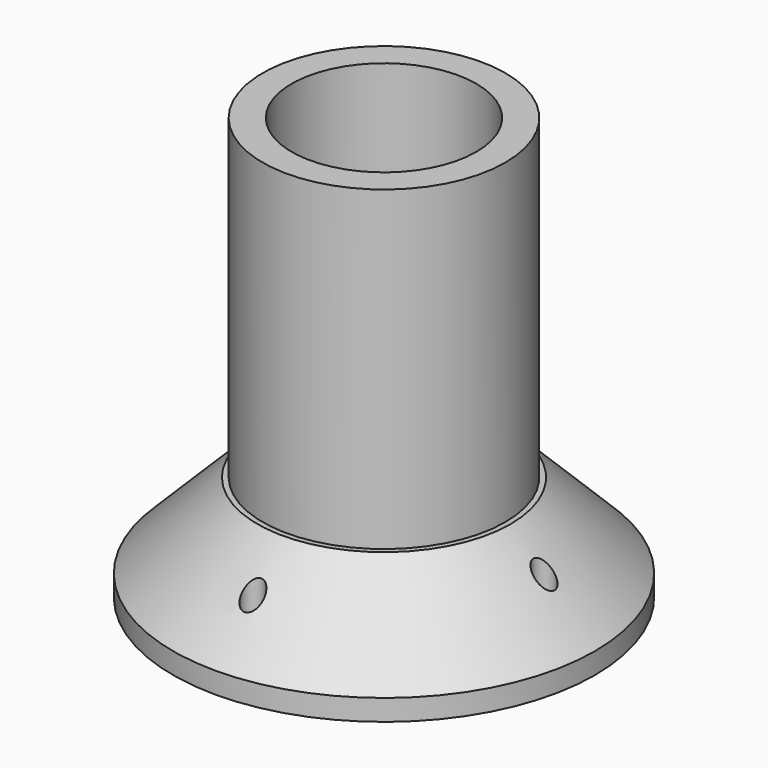
from build123d import *

# Parameters (mm, degrees)
F0_R     = 25.4
F0_R_2   = 1.27
F0_R_3   = 14.605
F1_DEPTH = 12.7
F0_R_4   = 11.1125
F2_DEPTH = 50.8


# Not quite as in the source:
# - a fillet or chamfer that OpenCascade refuses, or shapes differently, is made with other operations: its cross-section is extruded or revolved along the edge and cut away or added
# - a feature of the source that left no trace in its solid (it failed there, or was rolled back) is left out


with BuildPart() as f1:
    # F0 (on Top) → F1 (new body)
    with BuildSketch(Plane.XY):
        Circle(F0_R)
        with Locations((0, -19.7216775268)):
            Circle(F0_R_2, mode=Mode.SUBTRACT)
        with Locations((-19.3595029414, 0)):
            Circle(F0_R_2, mode=Mode.SUBTRACT)
        Circle(F0_R_3, mode=Mode.SUBTRACT)
        with Locations((19.2609746009, 0)):
            Circle(F0_R_2, mode=Mode.SUBTRACT)
        with Locations((0, 19.7912380099)):
            Circle(F0_R_2, mode=Mode.SUBTRACT)
    extrude(amount=F1_DEPTH)

    # F3: chamfer of 10.16 on 1 edges, made by hand

    # F3_s1 → F3_t2 (revolve, cut)
    with BuildSketch(Plane.XZ):
        Polygon((25.4, 2.54), (15.24, 12.7), (25.4, 12.7), align=None)
    revolve(axis=Axis((0, 0, 12.7), (0, 0, 1)), mode=Mode.SUBTRACT)


with BuildPart() as f2:
    # F0 (on Top) → F2 (new body)
    with BuildSketch(Plane.XY):
        Circle(F0_R_3)
        Circle(F0_R_4, mode=Mode.SUBTRACT)
    extrude(amount=F2_DEPTH)


solid = Compound([f1.part, f2.part])
